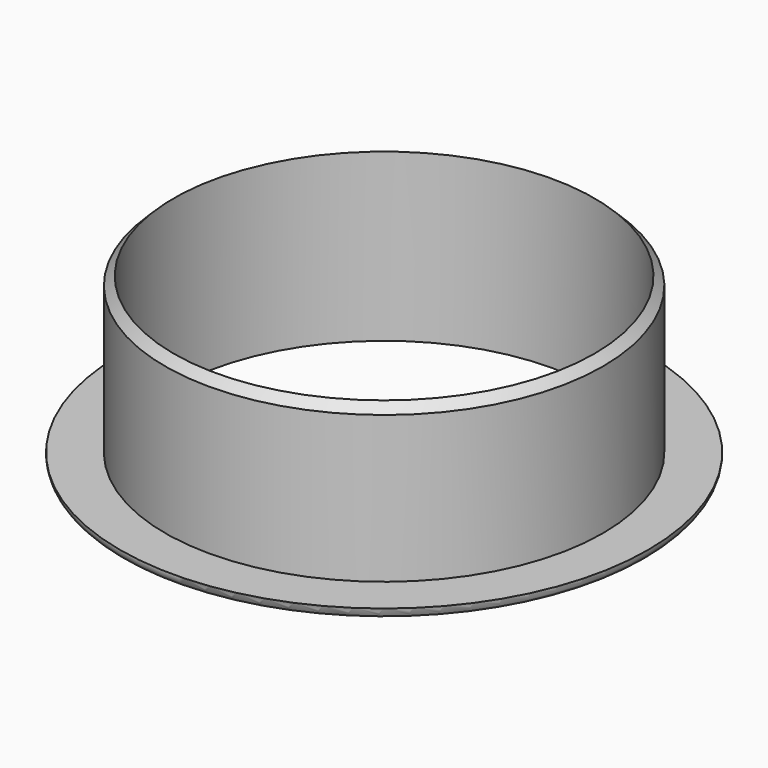
from build123d import *

# Parameters (mm, degrees)
F0_R     = 46.75
F0_R_2   = 38.75
F1_DEPTH = 2
F0_W     = 20
F0_H     = 24
F2_DEPTH = 30
F4_R     = 1.99999


# Not quite as in the source:
# - a fillet or chamfer that OpenCascade refuses, or shapes differently, is made with other operations: its cross-section is extruded or revolved along the edge and cut away or added
# - a fillet or chamfer is up to 0.001 mm smaller than in the source, because OpenCascade refuses the exact size


with BuildPart() as f1:
    # F0 (on Top) → F1 (new body)
    with BuildSketch(Plane.XY):
        Circle(F0_R)
        Circle(F0_R_2, mode=Mode.SUBTRACT)
    extrude(amount=F1_DEPTH)



with BuildPart() as f1b:
    # F0 (on Top) → F1, piece 2 (new body)
    with BuildSketch(Plane.XY):
        with BuildLine():
            ThreePointArc((-37.25, 0), (0, -37.25), (37.25, 0))
            Line((37.25, 0), (-37.25, 0))
        make_face()
        with Locations((0, -18.625)):
            Rectangle(F0_W, F0_H, mode=Mode.SUBTRACT)
    extrude(amount=F1_DEPTH)


with BuildPart() as f1_1:
    add(f1.part)

    add(f1b.part)  # F2 merges F1b
    # F0 (on Top) → F2 (join)
    with BuildSketch(Plane.XY):
        Circle(F0_R_2)
        with BuildLine():
            ThreePointArc((-37.25, 0), (0, 37.25), (37.25, 0))
            ThreePointArc((37.25, 0), (0, -37.25), (-37.25, 0))
        make_face(mode=Mode.SUBTRACT)
    extrude(amount=F2_DEPTH)

    # F3: chamfer of 2 on 1 edges, made by hand

    # F3_s1 → F3_t2 (revolve, cut)
    with BuildSketch(Plane.XZ):
        Polygon((36.75, 30), (38.75, 28), (38.75, 30), align=None)
    revolve(axis=Axis((0, 0, 30), (0, 0, 1)), mode=Mode.SUBTRACT)

    # F4 (radius 2 in the source; OpenCascade refuses exactly that, so slightly less here)
    f4_edges = [f1_1.edges().sort_by_distance(p)[0] for p in [
        (-46.75, 0, 0),
    ]]
    fillet(f4_edges, radius=F4_R)


solid = f1_1.part
